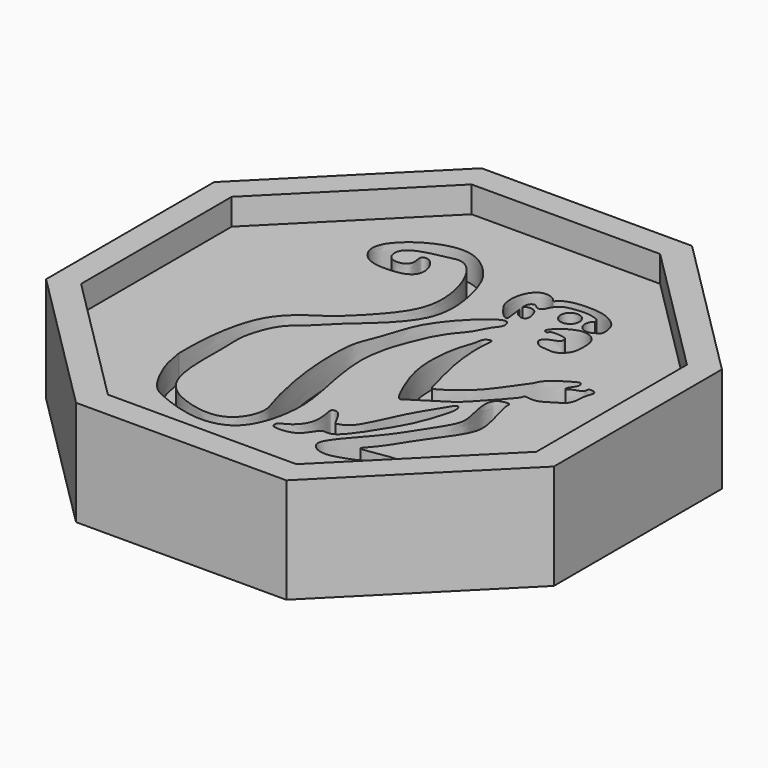
from build123d import *

# Parameters (mm, degrees)
F1_DEPTH = 25.4
F3_DEPTH = 6.35
F4_R     = 2.2716674016
F5_DEPTH = 6.35


with BuildPart() as f1:
    # F0 (on Top) → F1 (new body)
    with BuildSketch(Plane.XY):
        Polygon((-61.3372846899, 25.3607087968), (-61.3047391097, -25.4392807779), (-25.3607087968, -61.3372846899), (25.4392807779, -61.3047391097), (61.3372846899, -25.3607087968), (61.3047391097, 25.4392807779), (25.3607087968, 61.3372846899), (-25.4392807779, 61.3047391097), align=None)
    extrude(amount=F1_DEPTH)

    # F2 (on face) → F3 (cut)
    with BuildSketch(Plane.XY.offset(25.4)):
        Polygon((-54.9856008905, 22.734521413), (-54.9564255154, -22.8049569991), (-22.734521413, -54.9856008905), (22.8049569991, -54.9564255154), (54.9856008905, -22.734521413), (54.9564255154, 22.8049569991), (22.734521413, 54.9856008905), (-22.8049569991, 54.9564255154), align=None)
    extrude(amount=-F3_DEPTH, mode=Mode.SUBTRACT)

    # F4 (on face) → F5 (cut)
    with BuildSketch(Plane.XY.offset(19.05)):
        with BuildLine():
            add(Edge.make_bspline(
                [(-30.4572731256, -23.8665957004), (-30.1849697351, -25.471665321), (-29.7789483772, -29.2035450546), (-25.6413401126, -37.6312469304), (-21.2332613236, -39.7497742144), (-11.6026766248, -43.3255313967), (-1.2360447211, -40.8994420606), (1.8218766594, -27.3540267866), (0.0796147118, -18.0163368218), (-2.2491255985, -6.8231542093), (-1.3735615319, 2.0251338828), (1.1781596122, 7.9905515394), (2.4448321201, 10.8739295974)],
                knots=[0, 0, 0, 0, 0.0783055634, 0.1781599039, 0.2523690295, 0.3581767641, 0.4605394109, 0.5783071452, 0.6844463467, 0.79648054, 0.8964344897, 1, 1, 1, 1], degree=3))
            add(Edge.make_bspline(
                [(2.4448321201, 10.8739295974), (3.0778864816, 12.0437791866), (4.3686394261, 14.4290437746), (7.4390669956, 17.5004984115), (8.9003726766, 21.3337925752), (10.7808292686, 22.9749381329), (9.9161451921, 25.7282974423), (5.3493782343, 22.9974201056), (-2.5713572868, 14.414579051), (-4.1938414622, 6.8154161606), (-6.7320289767, 1.2899537383), (-7.5973672909, -2.7877695612), (-7.4939378882, -14.6064294224), (-4.6068217251, -27.6552075188), (-2.9169283324, -31.1470296944), (-3.9503947871, -35.9960998527), (-8.3064931178, -40.0964530822), (-16.9305838319, -38.9254526252), (-26.1795192673, -33.8065678679), (-24.8423451956, -16.0012345245), (-25.7498413573, -11.4361505347), (-23.0255360257, -2.9983883673), (-18.6917869218, -0.2512673239), (-14.8359516863, 4.1581994882), (-10.8403710107, 7.468038851), (-7.4145671758, 10.5789039926), (-0.130480085, 18.6454202492), (-2.6944553668, 31.8669637693), (-5.5315724864, 37.5838909793), (-11.6923987979, 43.0535652377), (-19.777570747, 42.3448953301), (-27.0465112615, 37.5596158979), (-29.7097735336, 32.3790997468), (-26.7888041645, 27.8821280577), (-21.7172966917, 27.2691291896), (-16.1391968629, 27.9199436825), (-14.5281434634, 31.4942051651), (-16.8535697651, 35.799239751), (-19.6049955957, 35.6648616321), (-18.9556901992, 33.5305638966), (-19.2468510655, 31.0116635304), (-23.8972561289, 30.6091075077), (-24.7890491057, 34.9148953778), (-21.278696336, 37.2288902151), (-15.9957994138, 38.1862198562), (-11.5448649575, 39.4899282186), (-6.7606592058, 33.9447351969), (-3.8071420804, 20.831471336), (-11.1710828952, 11.9321186611), (-16.8936723841, 6.034087606), (-22.0478031167, 3.1294473069), (-28.1023208606, -2.55639378), (-30.5004970595, -14.7723007569), (-30.4710025387, -20.9779337871), (-30.4572731256, -23.8665957004)],
                knots=[0, 0, 0, 0, 0.0156800401, 0.032028509, 0.0477955098, 0.0596958606, 0.0699204921, 0.08568389, 0.1127825607, 0.13490304, 0.1535116573, 0.1691480248, 0.1962756656, 0.2250379579, 0.2400645114, 0.2565053875, 0.2746038532, 0.2968928539, 0.3210059635, 0.3525368085, 0.3705019876, 0.3925531796, 0.4103376997, 0.4291317675, 0.4467336657, 0.4635817353, 0.4884670327, 0.5163134227, 0.5363602524, 0.5576529229, 0.5792980284, 0.6022487828, 0.6199788074, 0.6363257993, 0.6538828339, 0.6718081751, 0.6858642825, 0.702282458, 0.7126260492, 0.7229696404, 0.7345123922, 0.7491440131, 0.7630983917, 0.7781896689, 0.7966014056, 0.8123566002, 0.8320589901, 0.8599579659, 0.8859916596, 0.908273879, 0.9269981613, 0.948978231, 0.9762922978, 1, 1, 1, 1], degree=3))
        make_face()
        with BuildLine():
            add(Edge.make_bspline(
                [(6.6502266563, -23.9883847535), (6.9207478857, -23.6996770522), (8.7205427325, -23.5944244992), (10.3092368057, -28.1422955453), (11.0242948291, -27.7237907175), (14.0129990266, -26.9920531345), (17.1809222975, -18.9458853743), (20.7665480419, -12.6320803336), (22.9202332274, -9.3366033474), (24.0116511538, -7.4038169684), (25.1061801917, -8.8794213473), (24.1950817293, -12.7745215653), (22.1758373539, -18.4425552484), (19.6162778387, -22.8919706904), (16.2174019472, -28.3424692708), (12.7537249069, -32.3428354531), (10.0011312291, -31.105605123), (8.2969237725, -35.9181437869), (3.5885358873, -36.4170270791), (1.7806618488, -36.0872153415), (1.7587656793, -34.4059599168), (3.8866668084, -33.8791779188), (7.3423612882, -30.5807052492), (6.7524910513, -25.7470392599), (6.3806335274, -24.2761019604), (6.6502266563, -23.9883847535)],
                knots=[0, 0, 0, 0, 0.0299373702, 0.0794506071, 0.095630726, 0.1333004441, 0.2029541589, 0.2693198425, 0.3170805346, 0.3469409638, 0.3713742996, 0.4185061743, 0.4777647814, 0.5323108735, 0.5941117815, 0.6461214049, 0.6801310137, 0.7289151964, 0.7794452344, 0.8090712402, 0.8341373895, 0.8673716986, 0.9179812117, 0.9701653385, 1, 1, 1, 1], degree=3))
        make_face()
        with BuildLine():
            add(Edge.make_bspline(
                [(20.587073639, -32.7906049788), (20.5110411919, -32.4462974971), (22.9496121239, -30.1739076601), (25.9944237354, -24.9386152117), (28.7281349458, -21.0907434128), (33.2056993061, -14.9841617067), (33.8229461229, -10.4948583354), (30.9654812766, -2.3283066091), (31.5677879812, -0.8360378674), (27.0297102002, -1.2959121686), (28.0218097411, -7.6780092486), (29.4912886712, -12.3686166684), (26.0603233151, -17.6002396927), (21.5831526348, -24.8673660555), (17.4771130644, -29.3309519543), (14.935459807, -32.382826148), (11.9254741768, -36.4257715341), (15.36995079, -39.2478182958), (20.2555788817, -38.2951089492), (26.3100952478, -35.4935314276), (30.460662749, -33.471559903), (31.4592331037, -32.1986805363), (28.3818600714, -31.6541731038), (22.3842421061, -32.9187137138), (20.6385458557, -33.0236932189), (20.587073639, -32.7906049788)],
                knots=[0, 0, 0, 0, 0.0358239596, 0.0881161357, 0.1343534949, 0.1893783756, 0.2350599526, 0.294554235, 0.3145288723, 0.3493818407, 0.397862362, 0.4435960349, 0.4934417224, 0.5547153541, 0.6052599703, 0.6474299229, 0.6896762058, 0.7264981139, 0.77170675, 0.8266210464, 0.8709028571, 0.8901146479, 0.9216973173, 0.9757480039, 1, 1, 1, 1], degree=3))
        make_face()
        with BuildLine():
            add(Edge.make_bspline(
                [(10.5463499203, 14.5570253953), (10.6898119029, 15.2771527545), (10.6608859887, 16.49485645), (12.8696167357, 17.4022170374), (12.2014204751, 14.4831134954), (12.5417450658, 5.5758893193), (15.163696453, -3.0421764487), (15.5802482533, -5.7820800184), (18.4893945782, -4.058302174), (22.0537277652, -1.3879555458), (25.0444690292, 2.0379203743), (28.0198667208, 6.4927556934), (29.4688238969, 8.2462064281), (30.0492184898, 10.2834807423), (33.8954964575, 12.9373041208), (35.1795299498, 13.5412051897), (36.3919236597, 14.2850621551), (37.1644531853, 12.6829688658), (35.5350401829, 11.1536381285), (35.5468423805, 9.8359157056), (36.9652237321, 11.2229826588), (39.2974150976, 11.3762898063), (38.8706698255, 13.2955050651), (41.5218620232, 12.63739245), (40.2415397475, 10.7022401629), (40.3872210566, 8.0895953854), (39.663584398, 5.8426475888), (37.2984130339, 4.6769072022), (34.3085589144, 2.4620728683), (31.3583870418, 3.3977134953), (31.4473810927, 2.0523606954), (26.060168609, -3.3226645397), (23.1761527417, -7.0246769153), (15.4069967924, -11.189996312), (13.6614709622, -13.1974828199), (11.3723275887, -8.8328534054), (8.6941500703, -1.9273158202), (8.316938932, 4.6876565053), (9.1978015976, 10.9940583996), (10.3493781527, 13.5682982336), (10.5463499203, 14.5570253953)],
                knots=[0, 0, 0, 0, 0.0207787237, 0.0385975075, 0.0589652455, 0.105091958, 0.1510406189, 0.1709046067, 0.1946671679, 0.2270193885, 0.2596412707, 0.2941160722, 0.316113217, 0.3374737772, 0.3692352917, 0.388093052, 0.4034195226, 0.4196383883, 0.4418835035, 0.4543507383, 0.4725770781, 0.494295765, 0.5103188792, 0.5291877564, 0.5488390607, 0.5735046694, 0.5954384876, 0.6193169076, 0.6483341593, 0.6714783673, 0.6848128302, 0.7245515076, 0.7603608101, 0.8040801919, 0.8239535757, 0.8530932949, 0.8949676394, 0.9338657776, 0.9714710346, 1, 1, 1, 1], degree=3))
        make_face()
        with Locations((18.2830672711, 33.3343632519)):
            Circle(F4_R)
        with BuildLine():
            ThreePointArc((25.7887614948, 31.6651329885), (26.3205228323, 32.4255728482), (26.5079765663, 33.3343632519))
            ThreePointArc((26.5079765663, 33.3343632519), (25.2306053037, 35.3924507866), (22.8193983322, 35.1611877681))
            ThreePointArc((22.8193983322, 35.1611877681), (22.4608185553, 31.8475921246), (25.7887614948, 31.6651329885))
        make_face()
        with BuildLine():
            ThreePointArc((22.8193983322, 35.1611877681), (25.2306053037, 35.3924507866), (26.5079765663, 33.3343632519))
            ThreePointArc((26.5079765663, 33.3343632519), (26.3205228323, 32.4255728482), (25.7887614948, 31.6651329885))
            add(Edge.make_bspline(
                [(8.5621306401, 30.2359673893), (8.6707912569, 29.469641826), (8.8748005635, 28.0726522683), (8.9558573432, 27.0360002825), (9.1514699252, 25.4057839115), (7.3609805089, 26.6998171682), (6.2204486889, 28.2516065417), (4.6485538276, 30.1271595359), (4.5257350343, 34.4569171031), (6.117771848, 37.4005236371), (8.1832280029, 38.5772490208), (10.7370464933, 37.929515093), (11.4322938002, 36.5318850131), (12.0597348874, 37.6960278731), (14.402129811, 38.8114176636), (18.4024447036, 39.1387064997), (22.5699770857, 38.7059092357), (25.0490732437, 37.2186745895), (26.7032866039, 35.5859549895), (27.1466696778, 32.0905657234), (26.2650019211, 31.672651103), (25.7887614948, 31.6651329885)],
                knots=[0.3489172923, 0.3489172923, 0.3489172923, 0.3489172923, 0.3800474265, 0.4059920313, 0.4290794073, 0.4572949252, 0.4909018137, 0.5261626188, 0.5732532169, 0.6149026025, 0.6490610315, 0.685340708, 0.7092495181, 0.730251766, 0.7668889264, 0.8138513951, 0.8611448655, 0.89944325, 0.9347646888, 0.9753503008, 1, 1, 1, 1], degree=3))
            add(Edge.make_bspline(
                [(8.4240522527, 31.2757853698), (8.3354047683, 30.9953848673), (8.418932129, 30.6152306373), (8.5621306401, 30.2359673893)],
                knots=[0.7439152085, 0.7439152085, 0.7439152085, 0.7439152085, 0.8213951326, 0.8213951326, 0.8213951326, 0.8213951326], degree=3))
            add(Edge.make_bspline(
                [(22.8193983322, 35.1611877681), (22.84222454, 35.432872445), (22.877635586, 36.0462994886), (21.1041905044, 36.6817287138), (18.9829497241, 36.9926158134), (16.0697027851, 36.6770104597), (13.8358940291, 36.1518194947), (12.4157594107, 34.3186737894), (12.1972477866, 33.0953879645), (11.0275053497, 32.5465205215), (10.3085860216, 33.0934157122), (9.6596826084, 33.805098405), (8.3600064638, 32.9947929264), (8.3603372709, 31.880649559), (8.4240522527, 31.2757853698)],
                knots=[0, 0, 0, 0, 0.0198232021, 0.0492776657, 0.084082876, 0.1234920415, 0.1584104736, 0.192277645, 0.2175807613, 0.2412016347, 0.2622754424, 0.2831470152, 0.3089531787, 0.3346359236, 0.3346359236, 0.3346359236, 0.3346359236], degree=3))
        make_face()
        with BuildLine():
            add(Edge.make_bspline(
                [(9.6719777212, 28.4013785422), (10.027342167, 28.1176354995), (11.1063426805, 27.5616797843), (12.2139233125, 28.3988302967), (11.9153254201, 29.9465024236), (11.2972222158, 31.7179645863), (9.7213680989, 32.1122544658), (8.5642991902, 31.7193998954), (8.4240522527, 31.2757853698)],
                knots=[0, 0, 0, 0, 0.1275153677, 0.233307613, 0.3582635497, 0.4956064963, 0.621336185, 0.7439152085, 0.7439152085, 0.7439152085, 0.7439152085], degree=3))
            add(Edge.make_bspline(
                [(8.4240522527, 31.2757853698), (8.4454990704, 31.0721847153), (8.4928239903, 30.7266431786), (8.5424565779, 30.3747180913), (8.5621306401, 30.2359673893)],
                knots=[0.3346359236, 0.3346359236, 0.3346359236, 0.3346359236, 0.3432808785, 0.3489172923, 0.3489172923, 0.3489172923, 0.3489172923], degree=3))
            add(Edge.make_bspline(
                [(8.5621306401, 30.2359673893), (8.6943667935, 29.8857380984), (9.1514869475, 29.0133661724), (9.373629323, 28.6395967524), (9.6719777212, 28.4013785422)],
                knots=[0.8213951326, 0.8213951326, 0.8213951326, 0.8213951326, 0.8929436916, 1, 1, 1, 1], degree=3))
        make_face()
        with BuildLine():
            add(Edge.make_bspline(
                [(8.4240522527, 31.2757853698), (8.4454990704, 31.0721847153), (8.4928239903, 30.7266431786), (8.5424565779, 30.3747180913), (8.5621306401, 30.2359673893)],
                knots=[0.3346359236, 0.3346359236, 0.3346359236, 0.3346359236, 0.3432808785, 0.3489172923, 0.3489172923, 0.3489172923, 0.3489172923], degree=3))
            add(Edge.make_bspline(
                [(8.4240522527, 31.2757853698), (8.3354047683, 30.9953848673), (8.418932129, 30.6152306373), (8.5621306401, 30.2359673893)],
                knots=[0.7439152085, 0.7439152085, 0.7439152085, 0.7439152085, 0.8213951326, 0.8213951326, 0.8213951326, 0.8213951326], degree=3))
        make_face()
        with BuildLine():
            add(Edge.make_bspline(
                [(18.8456010073, 26.6272332519), (19.2281953217, 26.9188043779), (21.2092676023, 26.808091215), (23.1295492493, 26.4480806752), (22.8036113631, 24.6867960084), (20.9396300827, 24.3455711082), (19.9126590377, 23.6125024404), (18.9341053316, 22.6982114566), (20.4229753918, 20.8261720276), (22.3913901081, 20.8019169784), (25.0565899074, 20.3545999477), (27.1000358948, 22.4069828328), (27.6748326594, 24.3451816486), (27.6374354624, 28.1974720628), (26.4384213212, 29.8714363957), (23.9380274245, 30.9646444664), (20.9972068245, 29.9680772035), (18.5049367434, 28.1409990849), (17.3228298505, 26.2910419012), (18.6128105615, 25.9735958652), (18.6494707769, 26.4777644544), (18.8456010073, 26.6272332519)],
                knots=[0, 0, 0, 0, 0.0583602678, 0.1088608713, 0.1504450838, 0.2010836968, 0.2449306968, 0.2836888786, 0.336088855, 0.3899685898, 0.450928294, 0.5118310532, 0.5670306556, 0.6402347426, 0.6937559411, 0.7534839666, 0.8195821673, 0.8889460025, 0.9375916972, 0.9700826376, 1, 1, 1, 1], degree=3))
        make_face()
    extrude(amount=-F5_DEPTH, mode=Mode.SUBTRACT)


solid = f1.part
